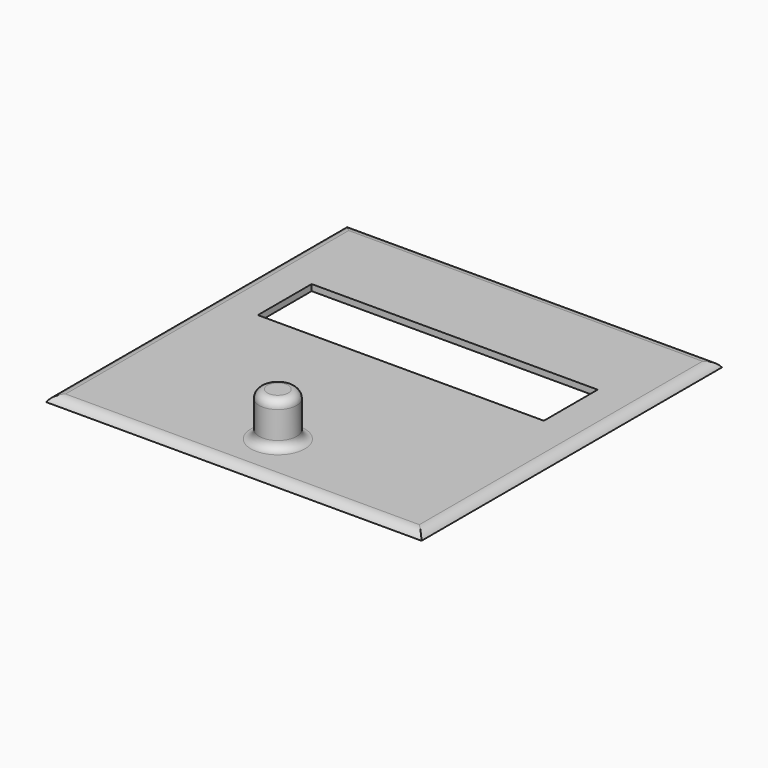
from build123d import *

# Parameters (mm, degrees)
F0_W          = 152.4
F0_H          = 2.54
F1_DEPTH      = 76.2
F1_DEPTH_BACK = 76.2
F2_W          = 116.0843670368
F2_H          = 27.2963345051
F3_DEPTH      = 25.4
F4_R          = 7.6032374963
F5_DEPTH      = 17.78
F6_R          = 3.3634669128
F7_T1_DEPTH   = 174.3970452561
F7_T3_DEPTH   = 174.3970452561


# Not quite as in the source:
# - a fillet or chamfer that OpenCascade refuses, or shapes differently, is made with other operations: its cross-section is extruded or revolved along the edge and cut away or added


with BuildPart() as f1:
    # F0 (on Front) → F1 (new body, two sides)
    with BuildSketch(Plane.XZ) as f1_sk:
        Rectangle(F0_W, F0_H)
    extrude(amount=-F1_DEPTH)
    extrude(f1_sk.sketch, amount=F1_DEPTH_BACK)

    # F2 (on face) → F3 (cut)
    with BuildSketch(Plane.XY.offset(1.27)):
        with Locations((0, 22.1970230341)):
            Rectangle(F2_W, F2_H)
    extrude(amount=-F3_DEPTH, mode=Mode.SUBTRACT)

    # F4 (on face) → F5 (join)
    with BuildSketch(Plane.XY.offset(1.27)):
        with Locations((0, -53.8427531719)):
            Circle(F4_R)
    extrude(amount=F5_DEPTH)

    # F6
    f6_edges = [f1.edges().sort_by_distance(p)[0] for p in [
        (7.603237, -53.842753, 10.16),
        (-7.603237, -53.842753, 1.27),
        (-7.603237, -53.842753, 19.05),
    ]]
    fillet(f6_edges, radius=F6_R)

    # F7: fillet of radius 5.08 on 4 edges, made by hand

    # F7_s2 → F7_t1 (cut)
    with BuildSketch(Plane.YZ.offset(-87.1985226281)):
        with BuildLine():
            ThreePointArc((-71.8005909488, 1.27), (-74.3405909488, 0.5894090512), (-76.2, -1.27))
            Line((-76.2, -1.27), (-76.2, 1.27))
            Line((-76.2, 1.27), (-71.8005909488, 1.27))
        make_face()
        with BuildLine():
            ThreePointArc((71.8005909488, 1.27), (74.3405909488, 0.5894090512), (76.2, -1.27))
            Line((76.2, -1.27), (76.2, 1.27))
            Line((76.2, 1.27), (71.8005909488, 1.27))
        make_face()
    extrude(amount=F7_T1_DEPTH, mode=Mode.SUBTRACT)

    # F7_s4 → F7_t3 (cut)
    with BuildSketch(Plane.XZ.offset(-87.1985226281)):
        with BuildLine():
            ThreePointArc((71.8005909488, 1.27), (74.3405909488, 0.5894090512), (76.2, -1.27))
            Line((76.2, -1.27), (76.2, 1.27))
            Line((76.2, 1.27), (71.8005909488, 1.27))
        make_face()
        with BuildLine():
            ThreePointArc((-71.8005909488, 1.27), (-74.3405909488, 0.5894090512), (-76.2, -1.27))
            Line((-76.2, -1.27), (-76.2, 1.27))
            Line((-76.2, 1.27), (-71.8005909488, 1.27))
        make_face()
    extrude(amount=F7_T3_DEPTH, mode=Mode.SUBTRACT)


solid = f1.part
